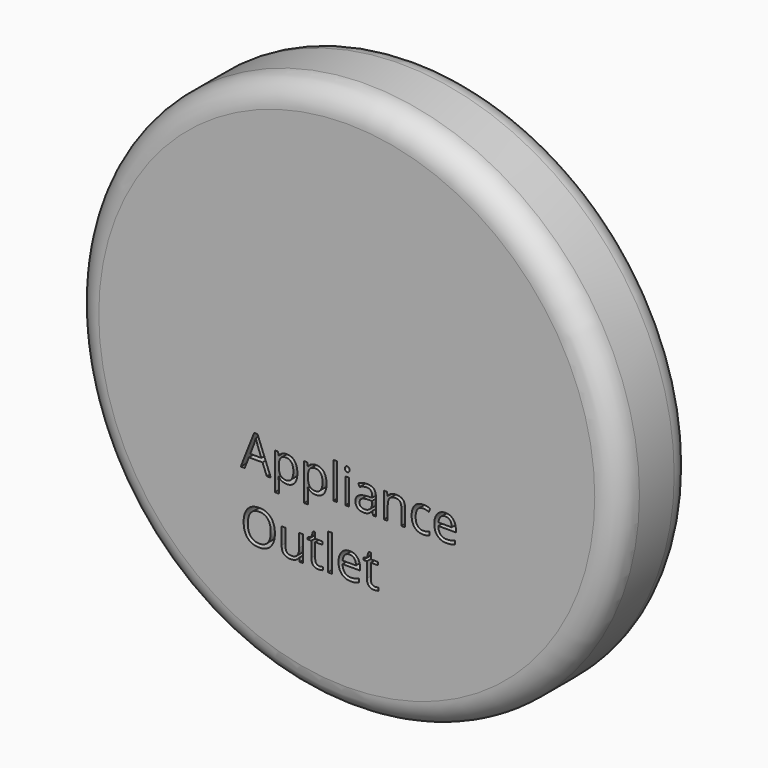
from build123d import *

# Parameters (mm, degrees)
F0_R         = 55.8317061579
F1_DEPTH     = 19.05
F2_R         = 5.08
F3_R         = 5.08
F4_TEXT_SIZE = 9.7424645598
F5_DEPTH     = 6.35


# Not quite as in the source:
# - Text() gives the source's letters only with a copy of the font that has no kerning and outlines rounded to 1/6400 em; it was checked with that copy


with BuildPart() as f1:
    # F0 (on Front) → F1 (new body)
    with BuildSketch(Plane.XZ):
        Circle(F0_R)
    extrude(amount=F1_DEPTH)

    # F2
    f2_edges = [f1.edges().sort_by_distance(p)[0] for p in [
        (-55.831706, -19.05, 0),
    ]]
    fillet(f2_edges, radius=F2_R)

    # F3
    f3_edges = [f1.edges().sort_by_distance(p)[0] for p in [
        (-55.831706, 0, 0),
    ]]
    fillet(f3_edges, radius=F3_R)

    # F4 (on face) → F5 (cut)
    with BuildSketch(Plane.XZ.offset(19.05)):
        with Locations((-21.7013433576, -18.0844515562)):
            Text('Appliance', F4_TEXT_SIZE, font='Open Sans', text_align=(TextAlign.LEFT, TextAlign.BOTTOM))
        with Locations((-21.7013433576, -31.3342033575)):
            Text('Outlet', F4_TEXT_SIZE, font='Open Sans', text_align=(TextAlign.LEFT, TextAlign.BOTTOM))
    extrude(amount=-F5_DEPTH, mode=Mode.SUBTRACT)


solid = f1.part
